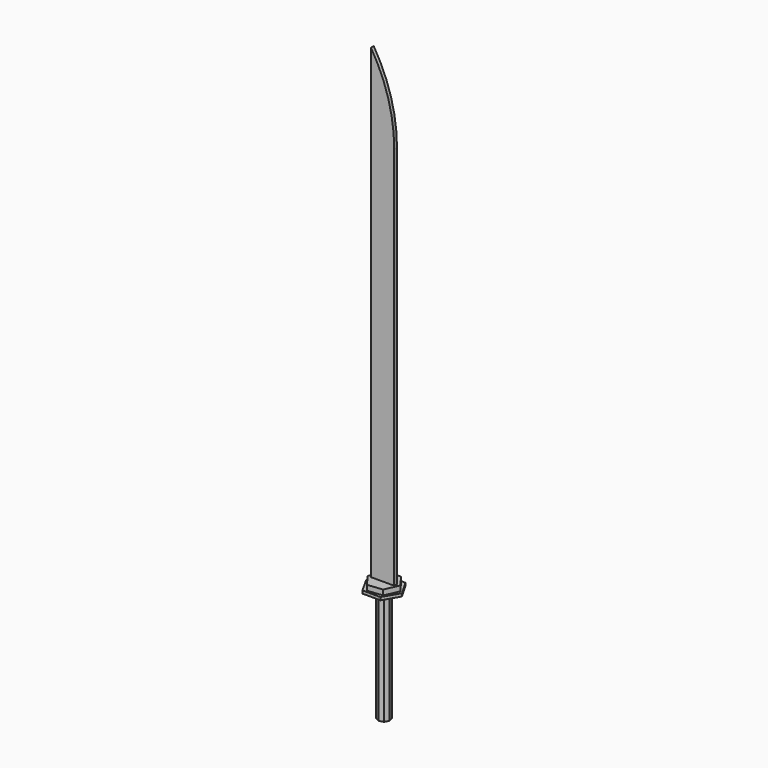
from build123d import *

# Parameters (mm, degrees)
F0_W        = 40.3080582619
F0_H        = 5.9715644456
F1_DEPTH    = 822
F3_DEPTH    = 196
F5_DEPTH    = 5
F6_T1_DEPTH = 716.1336390313
F8_DEPTH    = 14


# Not quite as in the source:
# - a fillet or chamfer that OpenCascade refuses, or shapes differently, is made with other operations: its cross-section is extruded or revolved along the edge and cut away or added


with BuildPart() as f1:
    # F0 (on Top) → F1 (new body)
    with BuildSketch(Plane.XY):
        Rectangle(F0_W, F0_H)
    extrude(amount=F1_DEPTH)

    # F2 (on Top) → F3 (join)
    with BuildSketch(Plane.XY):
        Polygon((6.5744029718, -8.407556447), (10.5938451005, -1.2962352533), (8.407556447, 6.5744029718), (1.2962352533, 10.5938451005), (-6.5744029718, 8.407556447), (-10.5938451005, 1.2962352533), (-8.407556447, -6.5744029718), (-1.2962352533, -10.5938451005), align=None)
    extrude(amount=-F3_DEPTH)

    # F4 (on Top) → F5 (join)
    with BuildSketch(Plane.XY):
        Polygon((31.1715127681, -0.1368859226), (15.7043030704, 26.9268789703), (-15.4672096977, 27.0637648929), (-31.1715127681, 0.1368859226), (-15.7043030704, -26.9268789703), (15.4672096977, -27.0637648929), align=None)
    extrude(amount=F5_DEPTH)

    # F6: fillet of radius 270.3919189858 on 1 edges, made by hand

    # F6_s2 → F6_t1 (cut)
    with BuildSketch(Plane.XZ.offset(-358.0668195157)):
        with BuildLine():
            ThreePointArc((-20.1540291309, 822), (9.881896476, 753.7882231999), (20.1540291309, 679.9675850829))
            Line((20.1540291309, 679.9675850829), (20.1540291309, 822))
            Line((20.1540291309, 822), (-20.1540291309, 822))
        make_face()
    extrude(amount=F6_T1_DEPTH, mode=Mode.SUBTRACT)

    # F7 (on face) → F8 (join)
    with BuildSketch(Plane(origin=(0, 0, 0), x_dir=(1, 0, 0), z_dir=(0, 0, -1))):
        Polygon((-10.5287277243, 23.8778866657), (-25.9432203033, 2.8207976541), (-15.4144925791, -21.0570890116), (10.5287277243, -23.8778866657), (25.9432203033, -2.8207976541), (15.4144925791, 21.0570890116), align=None)
    extrude(amount=-F8_DEPTH)


solid = f1.part
